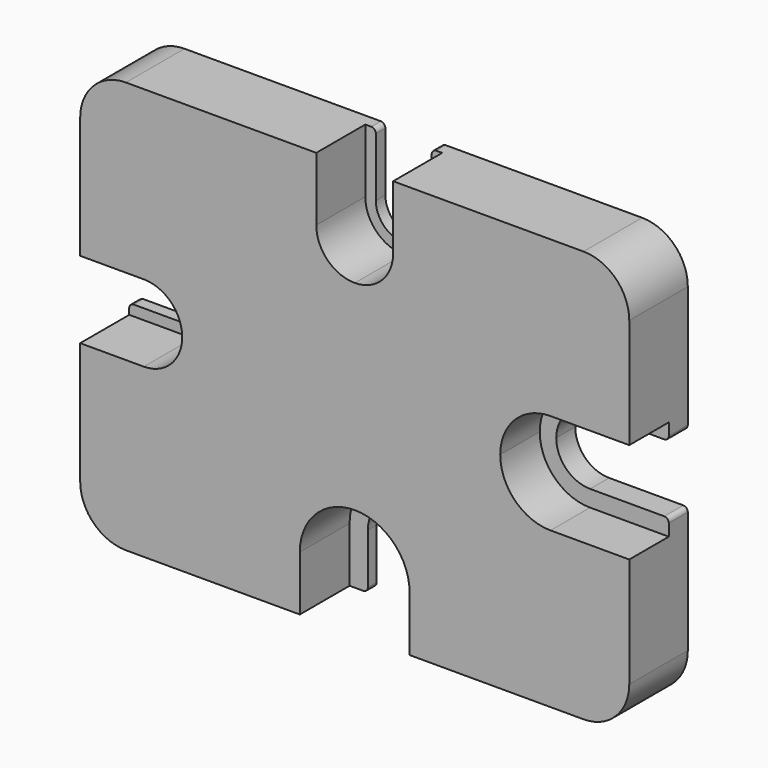
from build123d import *

# Parameters (mm, degrees)
F1_DEPTH = 8
F2_DEPTH = 1.3
F3_DEPTH = 2.6
F4_DEPTH = 1.3
F5_DEPTH = 1.2
F6_R     = 5
F7_R     = 0.5


with BuildPart() as f1:
    # F0 (on Front) → F1 (new body)
    with BuildSketch(Plane.XZ):
        with BuildLine():
            Line((6, -22.5), (30, -22.5))
            Line((30, -22.5), (30, -5.5))
            Line((30, -5.5), (21.4, -5.5))
            ThreePointArc((21.4, -5.5), (17.5109127035, -3.8890872965), (15.9, 0))
            ThreePointArc((15.9, 0), (17.5109127035, 3.8890872965), (21.4, 5.5))
            Line((21.4, 5.5), (30, 5.5))
            Line((30, 5.5), (30, 22.5))
            Line((30, 22.5), (4.2, 22.5))
            Line((4.2, 22.5), (4.2, 15.5500004172))
            ThreePointArc((4.2, 15.5500004172), (2.969848481, 12.5801519362), (0, 11.3500004172))
            ThreePointArc((0, 11.3500004172), (-2.969848481, 12.5801519362), (-4.2, 15.5500004172))
            Line((-4.2, 15.5500004172), (-4.2, 22.5))
            Line((-4.2, 22.5), (-30, 22.5))
            Line((-30, 22.5), (-30, 4.2))
            Line((-30, 4.2), (-23.05, 4.2))
            ThreePointArc((-23.05, 4.2), (-20.080151519, 2.969848481), (-18.85, 0))
            ThreePointArc((-18.85, 0), (-20.080151519, -2.969848481), (-23.05, -4.2))
            Line((-23.05, -4.2), (-30, -4.2))
            Line((-30, -4.2), (-30, -22.5))
            Line((-30, -22.5), (-6, -22.5))
            Line((-6, -22.5), (-6, -16.5))
            ThreePointArc((-6, -16.5), (-4.2426406871, -12.2573593129), (0, -10.5))
            ThreePointArc((0, -10.5), (4.2426406871, -12.2573593129), (6, -16.5))
            Line((6, -16.5), (6, -22.5))
        make_face()
    extrude(amount=F1_DEPTH)

    # F0 (on Front) → F2 (join)
    with BuildSketch(Plane.XZ):
        with BuildLine():
            Line((-30, -3.05), (-30, -4.2))
            Line((-30, -4.2), (-23.05, -4.2))
            ThreePointArc((-23.05, -4.2), (-20.080151519, -2.969848481), (-18.85, 0))
            ThreePointArc((-18.85, 0), (-20.080151519, 2.969848481), (-23.05, 4.2))
            Line((-23.05, 4.2), (-30, 4.2))
            Line((-30, 4.2), (-30, 3.05))
            Line((-30, 3.05), (-23.05, 3.05))
            ThreePointArc((-23.05, 3.05), (-20.8933243174, 2.1566756826), (-20, 0))
            ThreePointArc((-20, 0), (-20.8933243174, -2.1566756826), (-23.05, -3.05))
            Line((-23.05, -3.05), (-30, -3.05))
        make_face()
    extrude(amount=F2_DEPTH)

    # F0 (on Front) → F3 (join)
    with BuildSketch(Plane.XZ):
        with BuildLine():
            Line((21.4, -5.5), (30, -5.5))
            Line((30, -5.5), (30, -3.7))
            Line((30, -3.7), (21.4, -3.7))
            ThreePointArc((21.4, -3.7), (18.7837049096, -2.6162950904), (17.7, 0))
            ThreePointArc((17.7, 0), (18.7837049096, 2.6162950904), (21.4, 3.7))
            Line((21.4, 3.7), (30, 3.7))
            Line((30, 3.7), (30, 5.5))
            Line((30, 5.5), (21.4, 5.5))
            ThreePointArc((21.4, 5.5), (17.5109127035, 3.8890872965), (15.9, 0))
            ThreePointArc((15.9, 0), (17.5109127035, -3.8890872965), (21.4, -5.5))
        make_face()
    extrude(amount=F3_DEPTH)

    # F0 (on Front) → F4 (join)
    with BuildSketch(Plane.XZ):
        with BuildLine():
            Line((4.2, 15.5500004172), (4.2, 22.5))
            Line((4.2, 22.5), (3.05, 22.5))
            Line((3.05, 22.5), (3.05, 15.5500004172))
            ThreePointArc((3.05, 15.5500004172), (2.1566756826, 13.3933247346), (0, 12.5000004172))
            ThreePointArc((0, 12.5000004172), (-2.1566756826, 13.3933247346), (-3.05, 15.5500004172))
            Line((-3.05, 15.5500004172), (-3.05, 22.5))
            Line((-3.05, 22.5), (-4.2, 22.5))
            Line((-4.2, 22.5), (-4.2, 15.5500004172))
            ThreePointArc((-4.2, 15.5500004172), (-2.969848481, 12.5801519362), (0, 11.3500004172))
            ThreePointArc((0, 11.3500004172), (2.969848481, 12.5801519362), (4.2, 15.5500004172))
        make_face()
    extrude(amount=F4_DEPTH)

    # F0 (on Front) → F5 (join)
    with BuildSketch(Plane.XZ):
        with BuildLine():
            Line((4, -22.5), (6, -22.5))
            Line((6, -22.5), (6, -16.5))
            ThreePointArc((6, -16.5), (4.2426406871, -12.2573593129), (0, -10.5))
            ThreePointArc((0, -10.5), (-4.2426406871, -12.2573593129), (-6, -16.5))
            Line((-6, -16.5), (-6, -22.5))
            Line((-6, -22.5), (-4, -22.5))
            Line((-4, -22.5), (-4, -16.5))
            ThreePointArc((-4, -16.5), (-2.8284271247, -13.6715728753), (0, -12.5))
            ThreePointArc((0, -12.5), (2.8284271247, -13.6715728753), (4, -16.5))
            Line((4, -16.5), (4, -22.5))
        make_face()
    extrude(amount=F5_DEPTH)

    # F6
    f6_edges = [f1.edges().sort_by_distance(p)[0] for p in [
        (-30, -4, 22.5),
        (30, -4, 22.5),
        (-30, -4, -22.5),
        (30, -4, -22.5),
    ]]
    fillet(f6_edges, radius=F6_R)

    # F7
    f7_edges = [f1.edges().sort_by_distance(p)[0] for p in [
        (-30, -0.65, 3.05),
        (-30, -0.65, -3.05),
        (30, -1.3, 3.7),
        (30, -1.3, -3.7),
        (4, -0.6, -22.5),
        (-4, -0.6, -22.5),
        (3.05, -0.65, 22.5),
        (-3.05, -0.65, 22.5),
    ]]
    fillet(f7_edges, radius=F7_R)


solid = f1.part
